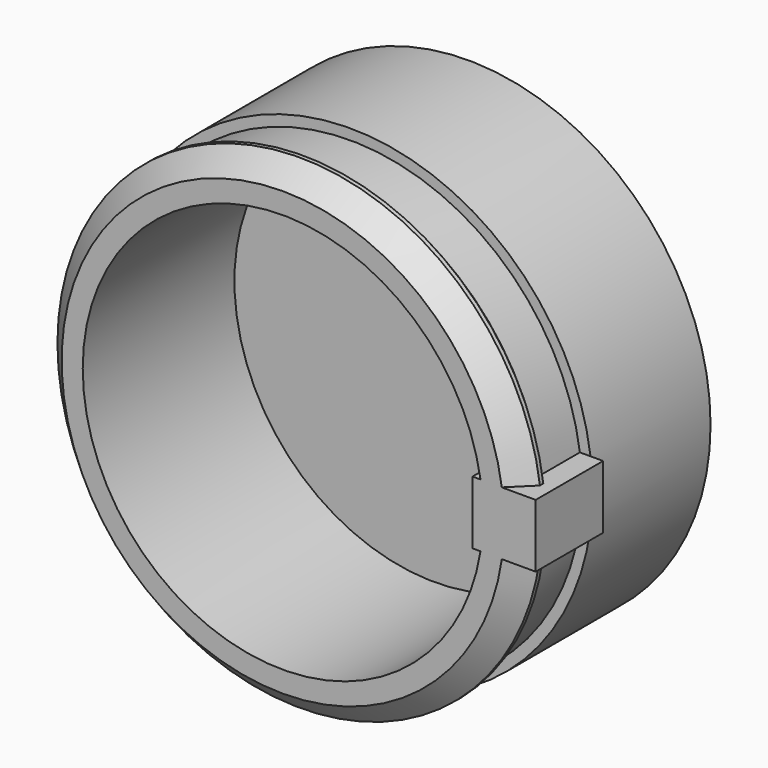
from build123d import *

# Parameters (mm, degrees)
F0_R        = 11.5
F0_R_2      = 9.5
F1_DEPTH    = 7
F2_DEPTH    = 2
F3_R        = 11
F3_R_2      = 9.5
F4_DEPTH    = 2
F5_R        = 11.5
F5_R_2      = 11
F5_R_3      = 9.5
F6_DEPTH    = 2
F7_S5_R     = 11
F7_T6_DEPTH = 18
F8_SIZE     = 1
F9_W        = 3
F9_H        = 3
F10_DEPTH   = 4


# Not quite as in the source:
# - a fillet or chamfer that OpenCascade refuses, or shapes differently, is made with other operations: its cross-section is extruded or revolved along the edge and cut away or added


with BuildPart() as f1:
    # F0 (on Front) → F1 (new body)
    with BuildSketch(Plane.XZ):
        Circle(F0_R)
        Circle(F0_R_2, mode=Mode.SUBTRACT)
    extrude(amount=F1_DEPTH)

    # F0 (on Front) → F2 (join)
    with BuildSketch(Plane.XZ):
        Circle(F0_R_2)
    extrude(amount=F2_DEPTH)

    # F3 (on face) → F4 (join)
    with BuildSketch(Plane.XZ.offset(7)):
        Circle(F3_R)
        Circle(F3_R_2, mode=Mode.SUBTRACT)
    extrude(amount=F4_DEPTH)

    # F5 (on face) → F6 (join)
    with BuildSketch(Plane.XZ.offset(9)):
        Circle(F5_R)
        Circle(F5_R_2, mode=Mode.SUBTRACT)
        Circle(F5_R_2)
        Circle(F5_R_3, mode=Mode.SUBTRACT)
    extrude(amount=F6_DEPTH)

    # F7: chamfer of 0.8 on 1 edges, made by hand


with BuildPart() as f7_tool2:
    # F7_s3 → F7_t4 (revolve)
    with BuildSketch(Plane.XY):
        Polygon((10.7, -9), (11.5, -9.8), (11.5, -9), align=None)
    revolve(axis=Axis((0, -9, 0), (0, -1, 0)))

    # F7_s5 → F7_t6 (cut, symmetric)
    with BuildSketch(Plane.XZ.offset(9.4)):
        Circle(F7_S5_R)
    extrude(amount=F7_T6_DEPTH, both=True, mode=Mode.SUBTRACT)


with BuildPart() as f1_1:
    add(f1.part)

    # F7_t1: cut F7_tool2
    add(f7_tool2.part, mode=Mode.SUBTRACT)

    # F8
    f8_edges = [f1_1.edges().sort_by_distance(p)[0] for p in [
        (-11.5, -11, 0),
    ]]
    chamfer(f8_edges, length=F8_SIZE)

    # F9 (on face) → F10 (join)
    with BuildSketch(Plane.XZ.offset(11)):
        with Locations((10.5, 0)):
            Rectangle(F9_W, F9_H)
    extrude(amount=-F10_DEPTH)


solid = f1_1.part
